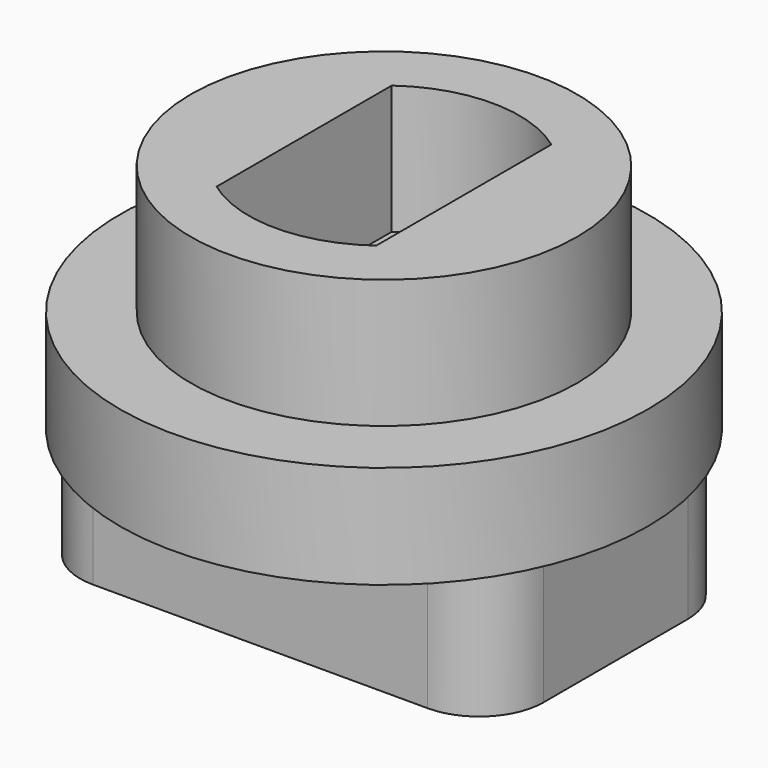
from build123d import *

# Parameters (mm, degrees)
F0_R         = 10.25
F1_DEPTH     = 4
F2_W         = 18
F2_H         = 12
F3_DEPTH     = 5
F4_W         = 15.4
F4_H         = 8.4
F5_DEPTH     = 5
F6_R         = 7.5
F7_DEPTH     = 5
F9_DEPTH     = 5
F10_T1_DEPTH = 11.25


# Not quite as in the source:
# - a fillet or chamfer that OpenCascade refuses, or shapes differently, is made with other operations: its cross-section is extruded or revolved along the edge and cut away or added


with BuildPart() as f1:
    # F0 (on Top) → F1 (new body)
    with BuildSketch(Plane.XY):
        Circle(F0_R)
    extrude(amount=F1_DEPTH)

    # F2 (on face) → F3 (join)
    with BuildSketch(Plane(origin=(0, 0, 0), x_dir=(1, 0, 0), z_dir=(0, 0, -1))):
        Rectangle(F2_W, F2_H)
    extrude(amount=F3_DEPTH)

    # F4 (on face) → F5 (cut)
    with BuildSketch(Plane(origin=(0, 0, -5), x_dir=(1, 0, 0), z_dir=(0, 0, -1))):
        Rectangle(F4_W, F4_H)
    extrude(amount=-F5_DEPTH, mode=Mode.SUBTRACT)

    # F6 (on face) → F7 (join)
    with BuildSketch(Plane.XY.offset(4)):
        Circle(F6_R)
    extrude(amount=F7_DEPTH)

    # F8 (on face) → F9 (cut)
    with BuildSketch(Plane.XY.offset(9)):
        with BuildLine():
            ThreePointArc((3.1, 4.25), (0, 5.2604657588), (-3.1, 4.25))
            Line((-3.1, 4.25), (-3.1, -4.25))
            ThreePointArc((-3.1, -4.25), (0, -5.2604657588), (3.1, -4.25))
            Line((3.1, -4.25), (3.1, 4.25))
        make_face()
    extrude(amount=-F9_DEPTH, mode=Mode.SUBTRACT)

    # F10: fillet of radius 2.5 on 4 edges, made by hand

    # F10_s2 → F10_t1 (cut)
    with BuildSketch(Plane.XY.offset(-11.25)):
        with BuildLine():
            ThreePointArc((-6.5, 6), (-8.267766953, 5.267766953), (-9, 3.5))
            Line((-9, 3.5), (-9, 6))
            Line((-9, 6), (-6.5, 6))
        make_face()
        with BuildLine():
            ThreePointArc((-9, -3.5), (-8.267766953, -5.267766953), (-6.5, -6))
            Line((-6.5, -6), (-9, -6))
            Line((-9, -6), (-9, -3.5))
        make_face()
        with BuildLine():
            ThreePointArc((9, -3.5), (8.267766953, -5.267766953), (6.5, -6))
            Line((6.5, -6), (9, -6))
            Line((9, -6), (9, -3.5))
        make_face()
        with BuildLine():
            ThreePointArc((9, 3.5), (8.267766953, 5.267766953), (6.5, 6))
            Line((6.5, 6), (9, 6))
            Line((9, 6), (9, 3.5))
        make_face()
    extrude(amount=F10_T1_DEPTH, mode=Mode.SUBTRACT)


solid = f1.part
